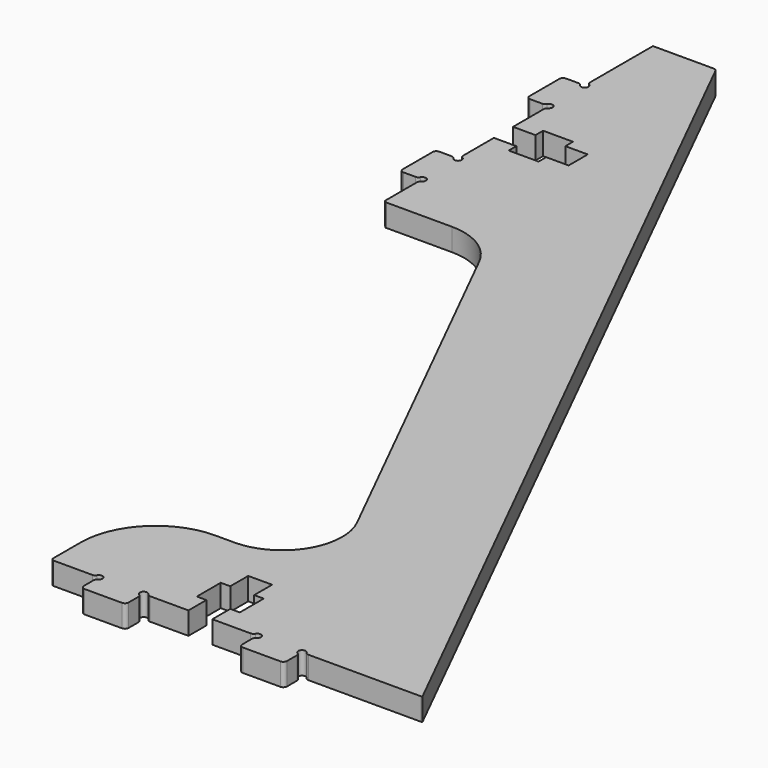
from build123d import *

# Parameters (mm, degrees)
F1_DEPTH = 3


# Not quite as in the source:
# - ends of sketch curves that miss each other by under 0.0002 mm in the source are joined


with BuildPart() as f1:
    # F0 (on Top) → F1 (new body)
    with BuildSketch(Plane.XY):
        with BuildLine():
            Line((-11.331514, -63.521951), (-6.04749, -63.521951))
            ThreePointArc((-6.04749, -63.521951), (-5.797538527, -63.4549610061), (-5.6145259066, -63.2719490539))
            ThreePointArc((-5.6145259066, -63.2719490539), (-4.8279591264, -63.1683980924), (-4.9315131291, -63.9549637764))
            ThreePointArc((-4.9315131291, -63.9549637764), (-5.1145256646, -64.1379759355), (-5.181513, -64.387976))
            Line((-5.181513, -64.387976), (-5.181517, -66.022003))
            ThreePointArc((-5.181517, -66.022003), (-5.0350703906, -66.3755563906), (-4.681517, -66.522003))
            Line((-4.681517, -66.522003), (0.318481, -66.522003))
            ThreePointArc((0.318481, -66.522003), (0.6720343906, -66.3755563906), (0.818481, -66.022003))
            Line((0.818481, -66.022003), (0.818481, -64.387974))
            ThreePointArc((0.818481, -64.387974), (0.7514940061, -64.137974527), (0.5684820539, -63.9549619066))
            ThreePointArc((0.5684820539, -63.9549619066), (0.4649300924, -63.1683971264), (1.2514957764, -63.2719511291))
            ThreePointArc((1.2514957764, -63.2719511291), (1.4345099355, -63.4549636646), (1.68451, -63.521951))
            Line((1.68451, -63.521951), (6.818481, -63.521951))
            Line((6.818481, -63.521951), (6.818481, -60.521979))
            Line((6.818481, -60.521979), (5.543485, -60.521979))
            Line((5.543485, -60.521979), (5.543485, -56.521951))
            Line((5.543485, -56.521951), (6.818481, -56.521951))
            Line((6.818481, -56.521951), (6.818481, -53.521951))
            Line((6.818481, -53.521951), (10.018491, -53.521951))
            Line((10.018491, -53.521951), (10.018491, -56.521951))
            Line((10.018491, -56.521951), (11.293485, -56.521951))
            Line((11.293485, -56.521951), (11.293485, -60.521979))
            Line((11.293485, -60.521979), (10.018491, -60.521979))
            Line((10.018491, -60.521979), (10.018491, -63.521951))
            Line((10.018491, -63.521951), (15.152465, -63.521948))
            ThreePointArc((15.152465, -63.521948), (15.4024642565, -63.4549611311), (15.5854768434, -63.2719494869))
            ThreePointArc((15.5854768434, -63.2719494869), (16.3720418736, -63.1683980924), (16.2684878709, -63.9549637764))
            ThreePointArc((16.2684878709, -63.9549637764), (16.0854743354, -64.1379759355), (16.018487, -64.387976))
            Line((16.018487, -64.387976), (16.018484, -66.022003))
            ThreePointArc((16.018484, -66.022003), (16.1649306094, -66.3755563906), (16.518484, -66.522003))
            Line((16.518484, -66.522003), (21.518482, -66.522003))
            ThreePointArc((21.518482, -66.522003), (21.8720353906, -66.3755563906), (22.018482, -66.022003))
            Line((22.018482, -66.022003), (22.018482, -64.387974))
            ThreePointArc((22.018482, -64.387974), (21.9514952226, -64.137974902), (21.7684838039, -63.9549623396))
            ThreePointArc((21.7684838039, -63.9549623396), (21.6649320924, -63.1683971264), (22.4514977764, -63.2719511291))
            ThreePointArc((22.4514977764, -63.2719511291), (22.634510152, -63.4549637896), (22.88451, -63.521951))
            Line((22.88451, -63.521951), (37.957041, -63.521951))
            ThreePointArc((37.957041, -63.521951), (38.0420573761, -63.4746028356), (38.0465663652, -63.3773953159))
            Line((38.0465663652, -63.3773953159), (-26.465295, 66.24561))
            ThreePointArc((-26.465295, 66.24561), (-26.6496426342, 66.4473285217), (-26.912508, 66.522003))
            Line((-26.912508, 66.522003), (-35.056991, 66.522003))
            Line((-35.056991, 66.522003), (-35.056987, 55.98807))
            ThreePointArc((-35.056987, 55.98807), (-34.9900000061, 55.738070527), (-34.8069880539, 55.5550579066))
            ThreePointArc((-34.8069880539, 55.5550579066), (-34.7034372218, 54.768492997), (-35.4900025264, 54.8720466961))
            ThreePointArc((-35.4900025264, 54.8720466961), (-35.6730149355, 55.0550596646), (-35.923015, 55.122047))
            Line((-35.923015, 55.122047), (-37.557041, 55.12205))
            ThreePointArc((-37.557041, 55.12205), (-37.9105943906, 54.9756033906), (-38.057041, 54.62205))
            Line((-38.057041, 54.62205), (-38.057041, 49.622052))
            ThreePointArc((-38.057041, 49.622052), (-37.9105943906, 49.2684986094), (-37.557041, 49.122052))
            Line((-37.557041, 49.122052), (-35.923013, 49.122052))
            ThreePointArc((-35.923013, 49.122052), (-35.673013527, 49.1890389939), (-35.4900009066, 49.3720509461))
            ThreePointArc((-35.4900009066, 49.3720509461), (-34.7034359497, 49.4756017309), (-34.8069901291, 48.6890362236))
            ThreePointArc((-34.8069901291, 48.6890362236), (-34.9900026646, 48.5060240645), (-35.05699, 48.256024))
            Line((-35.05699, 48.256024), (-35.05699, 43.122054))
            Line((-35.05699, 43.122054), (-32.057018, 43.122054))
            Line((-32.057018, 43.122054), (-32.057018, 44.397048))
            Line((-32.057018, 44.397048), (-28.05699, 44.397048))
            Line((-28.05699, 44.397048), (-28.05699, 43.122054))
            Line((-28.05699, 43.122054), (-25.05699, 43.122054))
            Line((-25.05699, 43.122054), (-25.05699, 39.922043))
            Line((-25.05699, 39.922043), (-28.05699, 39.922043))
            Line((-28.05699, 39.922043), (-28.05699, 38.647048))
            Line((-28.05699, 38.647048), (-32.057018, 38.647048))
            Line((-32.057018, 38.647048), (-32.057018, 39.922043))
            Line((-32.057018, 39.922043), (-35.05699, 39.922043))
            Line((-35.05699, 39.922043), (-35.056987, 34.788071))
            ThreePointArc((-35.056987, 34.788071), (-34.9900000061, 34.538071527), (-34.8069880539, 34.3550589066))
            ThreePointArc((-34.8069880539, 34.3550589066), (-34.7034372218, 33.568492997), (-35.4900025264, 33.6720466961))
            ThreePointArc((-35.4900025264, 33.6720466961), (-35.6730149355, 33.8550596646), (-35.923015, 33.922047))
            Line((-35.923015, 33.922047), (-37.557041, 33.92205))
            ThreePointArc((-37.557041, 33.92205), (-37.9105943906, 33.7756033906), (-38.057041, 33.42205))
            Line((-38.057041, 33.42205), (-38.057041, 28.422053))
            ThreePointArc((-38.057041, 28.422053), (-37.9105943906, 28.0684996094), (-37.557041, 27.922053))
            Line((-37.557041, 27.922053), (-35.923013, 27.922053))
            ThreePointArc((-35.923013, 27.922053), (-35.673013527, 27.9890399939), (-35.4900009066, 28.1720519461))
            ThreePointArc((-35.4900009066, 28.1720519461), (-34.7034359497, 28.2756027309), (-34.8069901291, 27.4890372236))
            ThreePointArc((-34.8069901291, 27.4890372236), (-34.9900026646, 27.3060250645), (-35.05699, 27.056025))
            Line((-35.05699, 27.056025), (-35.05699, 21.728049))
            Line((-35.05699, 21.728049), (-34.80699, 21.478049))
            Line((-34.80699, 21.478049), (-25.894542, 21.478049))
            ThreePointArc((-25.894542, 21.478049), (-21.6823966253, 20.2793600017), (-18.7325143305, 17.0425068355))
            Line((-18.7325143305, 17.0425068355), (8.142657, -36.957493))
            ThreePointArc((8.142657, -36.957493), (7.781941119, -44.7340961853), (0.98063, -48.521951))
            Line((0.98063, -48.521951), (-1.581514, -48.521951))
            ThreePointArc((-1.581514, -48.521951), (-8.6525818119, -51.4508831881), (-11.581514, -58.521951))
            Line((-11.581514, -58.521951), (-11.581514, -63.271951))
            Line((-11.581514, -63.271951), (-11.331514, -63.521951))
        make_face()
    extrude(amount=F1_DEPTH)


solid = f1.part
